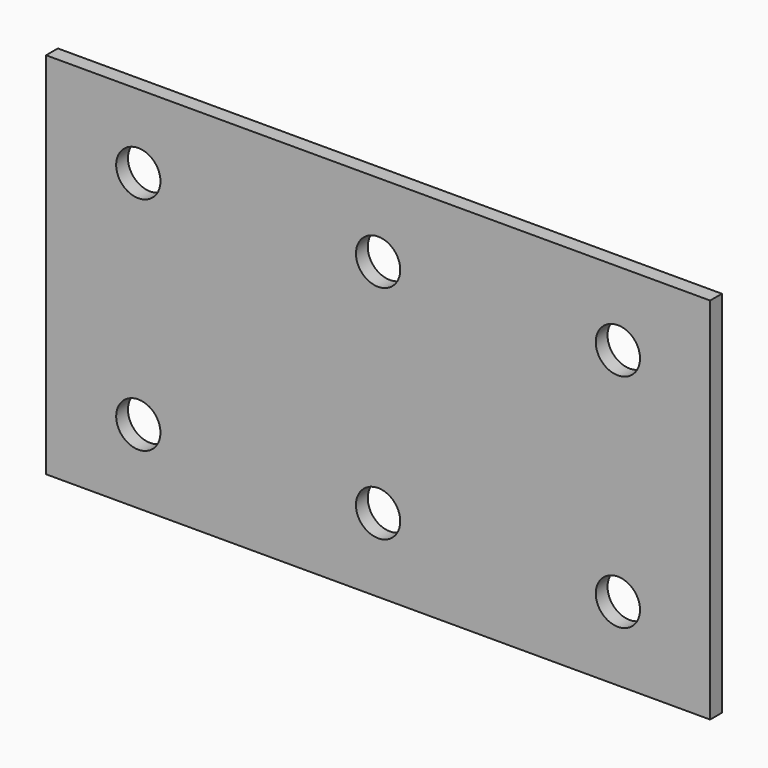
from build123d import *

# Parameters (mm, degrees)
F0_W     = 180
F0_H     = 100
F1_DEPTH = 4
F2_R     = 6
F3_R     = 6
F4_DEPTH = 100


with BuildPart() as f1:
    # F0 (on Front) → F1 (new body)
    with BuildSketch(Plane.XZ):
        with Locations((90, 50)):
            Rectangle(F0_W, F0_H)
    extrude(amount=F1_DEPTH)

    # F2 (on Front) + F3 (on face) → F4 (cut)
    with BuildSketch(Plane.XZ):
        with Locations((25, 80)):
            Circle(F2_R)
    with BuildSketch(Plane(origin=(0, 0, 0), x_dir=(-1, 0, 0), z_dir=(0, 1, 0))):
        with Locations((-155, 20)):
            Circle(F3_R)
        with Locations((-155, 80)):
            Circle(F3_R)
        with Locations((-25, 20)):
            Circle(F3_R)
        with Locations((-90, 80)):
            Circle(F3_R)
        with Locations((-90, 20)):
            Circle(F3_R)
    extrude(amount=F4_DEPTH, dir=(0, -1, 0), mode=Mode.SUBTRACT)


solid = f1.part
